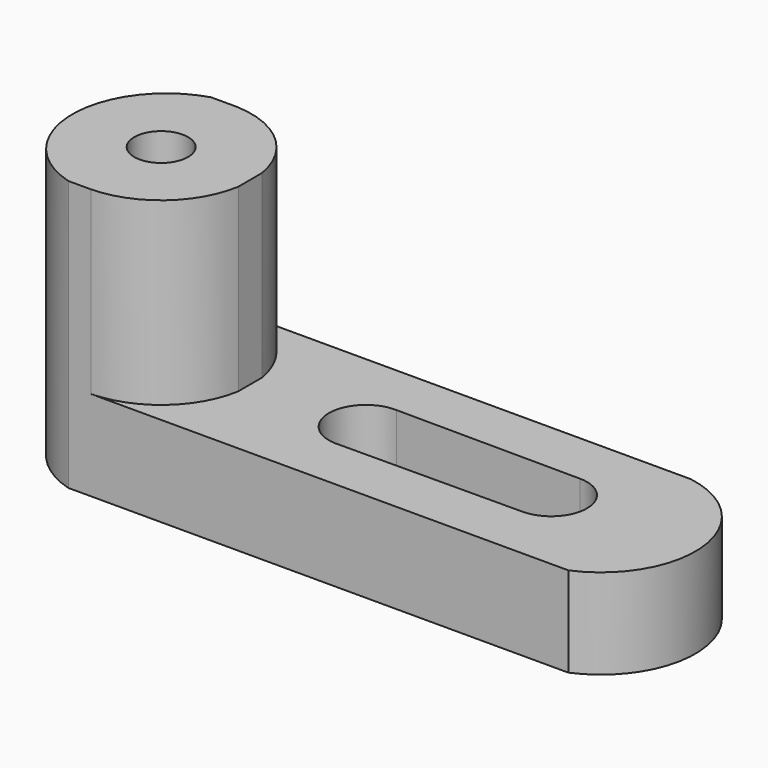
from build123d import *

# Parameters (mm, degrees)
F1_DEPTH  = 25.4
F3_DEPTH  = 25.4
F5_DEPTH  = 25.4
F7_DEPTH  = 25.4
F9_DEPTH  = 50.8
F13_DEPTH = 25.4
F14_R     = 3.8000451494
F15_DEPTH = 76.2
F17_DEPTH = 25.4


# Not quite as in the source:
# - the program builds the solid bodies; features that only make, move or delete a surface that nothing else refers to are left out


with BuildPart() as f1:
    # F0 (on Front) → F1 (new body)
    with BuildSketch(Plane.XZ):
        Polygon((-25.4, 38.1), (-25.4, 0), (63.5, 0), (63.5, 12.7), (0, 12.7), (0, 38.1), align=None)
    extrude(amount=F1_DEPTH)

    # F2 (on face) → F3 (cut)
    with BuildSketch(Plane.XZ.offset(25.4)):
        with BuildLine():
            ThreePointArc((-22.676864444, 0), (-24.571583371, 1.2835083224), (-25.4, 3.4168342035))
            Line((-25.4, 3.4168342035), (-25.4, 0))
            Line((-25.4, 0), (-22.676864444, 0))
        make_face()
    extrude(amount=-F3_DEPTH, mode=Mode.SUBTRACT)

    # F4 (on face) → F5 (cut)
    with BuildSketch(Plane.XY.offset(12.7)):
        with BuildLine():
            ThreePointArc((51.9632771611, 0), (63.0542215265, -11.5438688547), (55.0368912518, -25.4))
            Line((55.0368912518, -25.4), (63.5, -25.4))
            Line((63.5, -25.4), (63.5, 0))
            Line((63.5, 0), (51.9632771611, 0))
        make_face()
    extrude(amount=-F5_DEPTH, mode=Mode.SUBTRACT)

    # F6 (on face) → F7 (cut)
    with BuildSketch(Plane.XY.offset(38.1)):
        with BuildLine():
            ThreePointArc((-15.4641177505, -25.4), (-25.0669029781, -12.7718994312), (-15.6562179327, 0))
            Line((-15.6562179327, 0), (-25.4, 0))
            Line((-25.4, 0), (-25.4, -25.4))
            Line((-25.4, -25.4), (-15.4641177505, -25.4))
        make_face()
    extrude(amount=-F7_DEPTH, mode=Mode.SUBTRACT)

    # F8 (on face) → F9 (cut)
    with BuildSketch(Plane.XY.offset(12.7)):
        with BuildLine():
            Line((-25.4, 0), (-25.4, -25.4))
            Line((-25.4, -25.4), (-15.4641177505, -25.4))
            ThreePointArc((-15.4641177505, -25.4), (-25.0669029781, -12.7718994312), (-15.6562179327, 0))
            Line((-15.6562179327, 0), (-25.4, 0))
        make_face()
    extrude(amount=-F9_DEPTH, mode=Mode.SUBTRACT)

    # F12 (on face) → F13 (cut)
    with BuildSketch(Plane.XY.offset(38.1)):
        with BuildLine():
            ThreePointArc((-12.0063023642, 0), (-4.1167210002, -3.1788126596), (0, -10.6221286028))
            Line((0, -10.6221286028), (0, 0))
            Line((0, 0), (-12.0063023642, 0))
        make_face()
        with BuildLine():
            ThreePointArc((0, -14.7690480964), (-4.2265465157, -22.308409709), (-12.2979614132, -25.4))
            Line((-12.2979614132, -25.4), (0, -25.4))
            Line((0, -25.4), (0, -14.7690480964))
        make_face()
    extrude(amount=-F13_DEPTH, mode=Mode.SUBTRACT)

    # F14 (on face) → F15 (cut)
    with BuildSketch(Plane.XY.offset(38.1)):
        with Locations((-12.53633365, -12.6955883496)):
            Circle(F14_R)
    extrude(amount=-F15_DEPTH, mode=Mode.SUBTRACT)

    # F16 (on face) → F17 (cut)
    with BuildSketch(Plane.XY.offset(12.7)):
        with BuildLine():
            ThreePointArc((16.6168020143, -17.7693230367), (20.0435798879, -16.1217506564), (21.4334555491, -12.5826057047))
            ThreePointArc((21.4334555491, -12.5826057047), (19.9746784977, -8.9706846186), (16.4166737264, -7.3849335457))
            ThreePointArc((16.4166737264, -7.3849335457), (11.0325544335, -12.6828196506), (16.6168020143, -17.7693230367))
        make_face()
        with BuildLine():
            ThreePointArc((47.4116187176, -12.5826057047), (45.9414348271, -9.0192691511), (42.3863259992, -7.5292995919))
            ThreePointArc((42.3863259992, -7.5292995919), (37.304850424, -12.5816406618), (42.3843959412, -17.6359221781))
            ThreePointArc((42.3843959412, -17.6359221781), (45.9407542727, -16.1466264756), (47.4116187176, -12.5826057047))
        make_face()
        with BuildLine():
            ThreePointArc((16.4166737264, -7.3849335457), (19.9746784977, -8.9706846186), (21.4334555491, -12.5826057047))
            ThreePointArc((21.4334555491, -12.5826057047), (20.0435798879, -16.1217506564), (16.6168020143, -17.7693230367))
            Line((16.6168020143, -17.7693230367), (42.3843959412, -17.6359221781))
            ThreePointArc((42.3843959412, -17.6359221781), (37.304850424, -12.5816406618), (42.3863259992, -7.5292995919))
            Line((42.3863259992, -7.5292995919), (16.4166737264, -7.3849335457))
        make_face()
    extrude(amount=-F17_DEPTH, mode=Mode.SUBTRACT)


solid = f1.part
